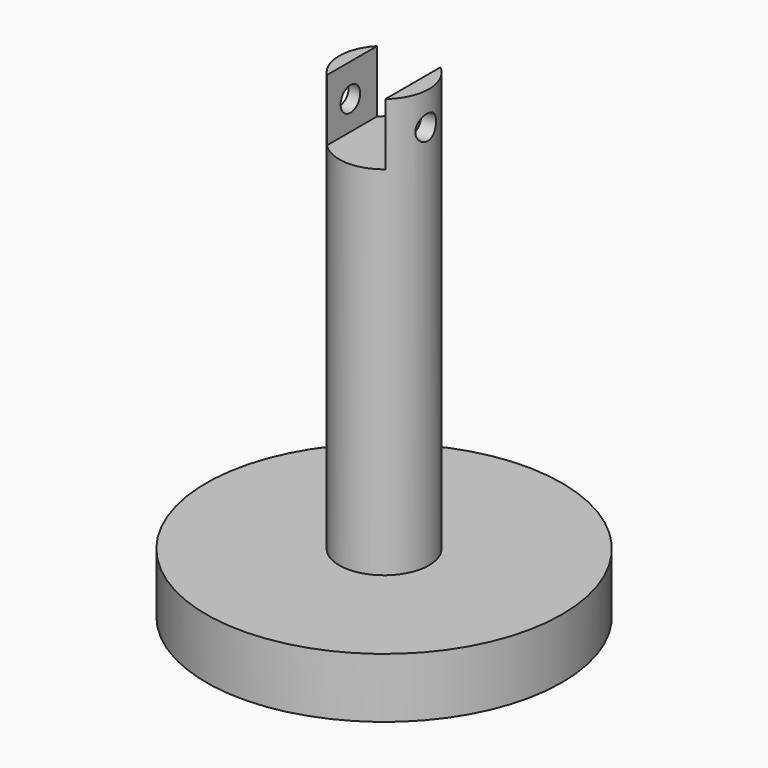
from build123d import *

# Parameters (mm, degrees)
F0_R     = 75.4315959701
F1_DEPTH = 25.4
F10_R    = 19.05
F2_DEPTH = 203.2
F4_DEPTH = 26.25509
F5_R     = 5.3383463792
F6_DEPTH = 25.4
F7_R     = 5.1969918097
F8_DEPTH = 22.39609
F9_DEPTH = 72.38519


# Not quite as in the source:
# - a feature names something its author has since deleted; it is built from what else it names


with BuildPart() as f1:
    # F0 (on Top) → F1 (new body)
    with BuildSketch(Plane.XY):
        Circle(F0_R)
    extrude(amount=F1_DEPTH)

    # F10 (on Top) → F2 (join)
    with BuildSketch(Plane.XY):
        Circle(F10_R)
    extrude(amount=F2_DEPTH)

    # F3 (on face) → F4 (cut)
    with BuildSketch(Plane.XY.offset(203.2)):
        with BuildLine():
            ThreePointArc((12.2368524888, 14.6000664782), (-0.9386041951, 19.026863172), (-13.6144, 13.3248119176))
            Line((-13.6144, 13.3248119176), (-13.6144, -13.3248119176))
            ThreePointArc((-13.6144, -13.3248119176), (-0.9386041951, -19.026863172), (12.2368524888, -14.6000664782))
            Line((12.2368524888, -14.6000664782), (12.2368524888, 14.6000664782))
        make_face()
    extrude(amount=-F4_DEPTH, mode=Mode.SUBTRACT)

    # F5 (on face) → F6 (cut)
    with BuildSketch(Plane.YZ.offset(-13.6144)):
        with Locations((-189.9197250605, 0)):
            Circle(F5_R)
    extrude(amount=-F6_DEPTH, mode=Mode.SUBTRACT)

    # F7 (on face) → F8 (cut)
    with BuildSketch(Plane.YZ.offset(-13.6144)):
        with Locations((-0.8483366109, 189.2552375793)):
            Circle(F7_R)
    extrude(amount=-F8_DEPTH, mode=Mode.SUBTRACT)

    # F7 (on face) → F9 (cut)
    with BuildSketch(Plane.YZ.offset(-13.6144)):
        with Locations((-0.8483366109, 189.2552375793)):
            Circle(F7_R)
    extrude(amount=F9_DEPTH, mode=Mode.SUBTRACT)


solid = f1.part
